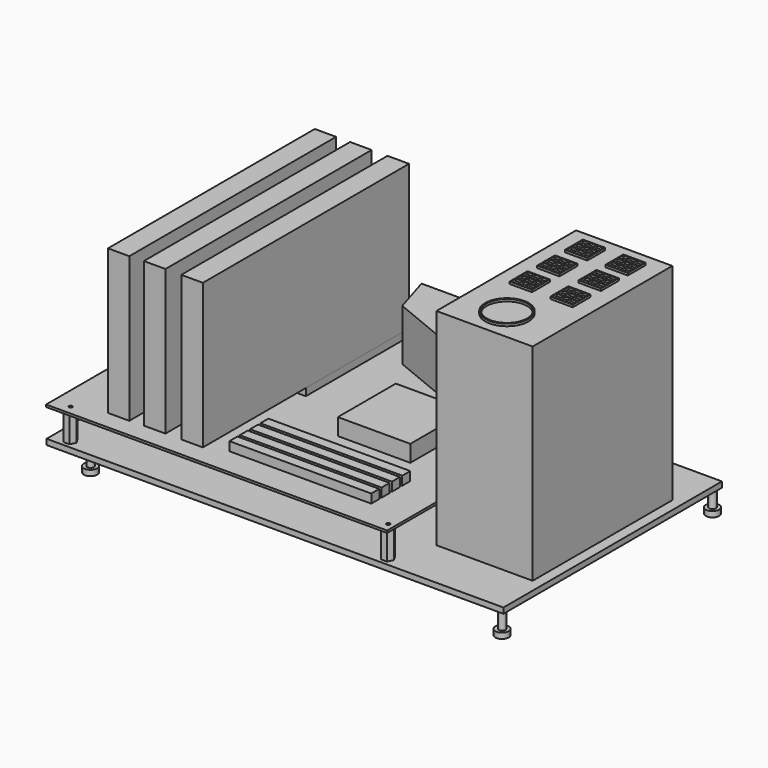
from build123d import *

# Parameters (mm, degrees)
F0_W      = 304.8
F0_H      = 245
F0_W_2    = 105
F0_W_3    = 85
F0_H_2    = 155
F1_DEPTH  = 5
F2_R      = 2
F4_DEPTH  = 25
F5_W      = 305.9651181102
F5_H      = 238.5258898139
F5_R      = 1.5110835086
F5_R_2    = 1.8546017652
F5_R_3    = 1.5453334322
F5_R_4    = 1.5864873671
F5_R_5    = 1.5329396313
F5_R_6    = 1.5189337909
F6_DEPTH  = 2
F8_DEPTH  = 46
F9_W      = 86.2980593292
F9_H      = 156.6275962591
F10_DEPTH = 185
F11_R     = 19.4404992454
F11_R_2   = 18.1570316282
F11_W     = 20
F11_H     = 20
F11_W_2   = 5.8072507381
F11_H_2   = 5.6268667936
F11_H_3   = 5.6345332414
F11_W_3   = 5.6646615267
F11_W_4   = 5.666539073
F11_W_5   = 5.6
F11_H_4   = 5.6
F11_W_6   = 5.645275116
F11_H_5   = 5.608684849
F12_DEPTH = 2
F7_W      = 10.3331357241
F7_H      = 111.6103834684
F7_W_2    = 9.9950507283
F7_H_2    = 111.5762374575
F7_H_3    = 111.7404969409
F13_DEPTH = 7
F14_W     = 19.3574428558
F14_H     = 231.2334789895
F14_W_2   = 10.3331357241
F14_H_2   = 111.6103834684
F14_W_3   = 19.1079676151
F14_H_3   = 231.8987650797
F15_DEPTH = 130
F7_W_3    = 65
F7_H_4    = 65
F16_DEPTH = 15
F7_W_4    = 127.2524446249
F7_H_5    = 8.9775174856
F17_DEPTH = 8
F18_R     = 3
F19_DEPTH = 15
F20_R     = 6
F21_DEPTH = 5


# Not quite as in the source:
# - a feature names something its author has since deleted; it is built from what else it names


with BuildPart() as f1:
    # F0 (on Top) → F1 (new body)
    with BuildSketch(Plane.XY):
        with Locations((-82.8795462154, -8.5489067304)):
            Rectangle(F0_W, F0_H)
        Polygon((-217.9899460981, -119.0375398017), (-216.8253733572, -121.0318073611), (-215.6608004927, -123.0260751322), (-216.8056005272, -125.0317585543), (-217.95040061, -127.0374420608), (-220.2597738008, -127.0488578615), (-222.5691463327, -127.060273659), (-223.7337190736, -125.0660060997), (-224.8982919382, -123.0717383286), (-223.7534917181, -121.0660545815), (-222.6086918209, -119.0603714), (-220.2993194058, -119.0489556031), align=None, mode=Mode.SUBTRACT)
        Polygon((-90.5598577739, -62.1443010035), (-89.4611932931, -64.1756228432), (-88.3625285496, -66.2069451687), (-89.5723726919, -68.1740775467), (-90.7822169912, -70.14121018), (-93.0907256892, -70.0770206068), (-95.399234657, -70.0128310261), (-96.4978992478, -67.9815089828), (-97.5965638812, -65.9501868608), (-96.386719739, -63.9830544828), (-95.1768754397, -62.0159218495), (-92.8683667417, -62.0801114227), align=None, mode=Mode.SUBTRACT)
        Polygon((68.33831607, -120.4494335332), (68.5094554206, -122.7524848222), (68.6805947525, -125.0555358592), (66.7716636058, -126.3552724604), (64.862732467, -127.6550090563), (62.7826618455, -126.6516944255), (60.7025914991, -125.6483799275), (60.5314521485, -123.3453286385), (60.3603128167, -121.0422776016), (62.2692441546, -119.7425408701), (64.1781751021, -118.4428044045), (66.2582453863, -119.4461188725), align=None, mode=Mode.SUBTRACT)
        Polygon((66.8298548613, -49.0489067304), (67.9845552805, -51.048906524), (69.1392559381, -53.0489067304), (67.9845553961, -55.0489067366), (66.8298548613, -57.0489067304), (64.5204537846, -57.0489067304), (62.2110527078, -57.0489067304), (61.0563521016, -55.0489066128), (59.9016516311, -53.0489067304), (61.056352173, -51.0489067242), (62.2110527078, -49.0489067304), (64.5204537846, -49.0489067304), align=None, mode=Mode.SUBTRACT)
        Polygon((-214.9167182465, 106.9143115381), (-213.840469393, 104.871024627), (-212.7642204714, 102.8277375865), (-213.9956343223, 100.8740354331), (-215.2270484403, 98.9203328559), (-217.5347112225, 99.0099174629), (-219.8423741843, 99.0995020768), (-220.9186230378, 101.1427889879), (-221.9948719595, 103.1860760283), (-220.7634577856, 105.1397786942), (-219.5320439906, 107.093480759), (-217.2243815961, 107.003896167), align=None, mode=Mode.SUBTRACT)
        Polygon((-90.6970964333, 107.0223465499), (-89.5289724143, 105.0301567779), (-88.3608485, 103.0379671844), (-89.5020735318, 101.0302470656), (-90.6432982822, 99.022527442), (-92.9526471492, 99.0069972534), (-95.2619959976, 98.991467065), (-96.4301198271, 100.9836565138), (-97.5982439308, 102.9758464304), (-96.4570190841, 104.9835662237), (-95.3157941487, 106.9912861729), (-93.0064452817, 107.0068163614), align=None, mode=Mode.SUBTRACT)
        Polygon((66.8699328729, 82.7181310753), (67.9002257868, 81.0905187095), (68.9305187879, 79.462906206), (68.3003771909, 77.6425906742), (67.6702358065, 75.8222757565), (65.8541689997, 75.1799921406), (64.0381027187, 74.5377087107), (62.4036458006, 75.5571097754), (60.7691898217, 76.5765102543), (60.5471225276, 78.4899656062), (60.3250552006, 80.4034212412), (61.6825983651, 81.770060566), (63.0401412837, 83.1366996433), (64.9550370207, 82.9274153656), align=None, mode=Mode.SUBTRACT)
        with Locations((122.0204537846, -8.5489067304)):
            Rectangle(F0_W_2, F0_H)
        with Locations((122.0204537846, -8.5489067304)):
            Rectangle(F0_W_3, F0_H_2, mode=Mode.SUBTRACT)
        with BuildLine():
            ThreePointArc((62.2692441546, -119.7425408701), (64.2240317575, -119.0599051032), (66.2582453863, -119.4461188725))
            Line((66.2582453863, -119.4461188725), (64.1781751021, -118.4428044045))
            Line((64.1781751021, -118.4428044045), (62.2692441546, -119.7425408701))
        make_face()
        with BuildLine():
            ThreePointArc((60.5314521485, -123.3453286385), (60.9176661018, -121.3111147656), (62.2692441546, -119.7425408701))
            Line((62.2692441546, -119.7425408701), (60.3603128167, -121.0422776016))
            Line((60.3603128167, -121.0422776016), (60.5314521485, -123.3453286385))
        make_face()
        with BuildLine():
            Line((64.862732467, -127.6550090563), (66.7716636058, -126.3552724604))
            ThreePointArc((66.7716636058, -126.3552724604), (64.8168757402, -127.0379083629), (62.7826618455, -126.6516944255))
            Line((62.7826618455, -126.6516944255), (64.862732467, -127.6550090563))
        make_face()
        with BuildLine():
            ThreePointArc((68.5094554206, -122.7524848222), (68.5177032479, -122.9005937913), (68.5204537846, -123.0489067304))
            ThreePointArc((68.5204537846, -123.0489067304), (68.0563298631, -124.9190886353), (66.7716636058, -126.3552724604))
            Line((66.7716636058, -126.3552724604), (68.6805947525, -125.0555358592))
            Line((68.6805947525, -125.0555358592), (68.5094554206, -122.7524848222))
        make_face()
        with BuildLine():
            Line((60.7025914991, -125.6483799275), (62.7826618455, -126.6516944255))
            ThreePointArc((62.7826618455, -126.6516944255), (61.2140879787, -125.3001164402), (60.5314521485, -123.3453286385))
            Line((60.5314521485, -123.3453286385), (60.7025914991, -125.6483799275))
        make_face()
        with BuildLine():
            ThreePointArc((66.2582453863, -119.4461188725), (67.8268194851, -120.7976968657), (68.5094554206, -122.7524848222))
            Line((68.5094554206, -122.7524848222), (68.33831607, -120.4494335332))
            Line((68.33831607, -120.4494335332), (66.2582453863, -119.4461188725))
        make_face()
        with BuildLine():
            ThreePointArc((-92.8683667417, -62.0801114227), (-90.8840347309, -62.6713924621), (-89.4611932931, -64.1756228432))
            Line((-89.4611932931, -64.1756228432), (-90.5598577739, -62.1443010035))
            Line((-90.5598577739, -62.1443010035), (-92.8683667417, -62.0801114227))
        make_face()
        with BuildLine():
            ThreePointArc((-96.386719739, -63.9830544828), (-94.8824892694, -62.5602130289), (-92.8683667417, -62.0801114227))
            Line((-92.8683667417, -62.0801114227), (-95.1768754397, -62.0159218495))
            Line((-95.1768754397, -62.0159218495), (-96.386719739, -63.9830544828))
        make_face()
        with BuildLine():
            ThreePointArc((-96.4978992478, -67.9815089828), (-96.9780008064, -65.9673865034), (-96.386719739, -63.9830544828))
            Line((-96.386719739, -63.9830544828), (-97.5965638812, -65.9501868608))
            Line((-97.5965638812, -65.9501868608), (-96.4978992478, -67.9815089828))
        make_face()
        with BuildLine():
            Line((-95.399234657, -70.0128310261), (-93.0907256892, -70.0770206068))
            ThreePointArc((-93.0907256892, -70.0770206068), (-95.0750577985, -69.4857395068), (-96.4978992478, -67.9815089828))
            Line((-96.4978992478, -67.9815089828), (-95.399234657, -70.0128310261))
        make_face()
        with BuildLine():
            Line((-90.7822169912, -70.14121018), (-89.5723726919, -68.1740775467))
            ThreePointArc((-89.5723726919, -68.1740775467), (-91.0766031615, -69.5969190007), (-93.0907256892, -70.0770206068))
            Line((-93.0907256892, -70.0770206068), (-90.7822169912, -70.14121018))
        make_face()
        with BuildLine():
            ThreePointArc((-89.4611932931, -64.1756228432), (-89.1018270605, -65.0970905156), (-88.9795462154, -66.0785660148))
            ThreePointArc((-88.9795462154, -66.0785660148), (-89.1306051861, -67.1674429375), (-89.5723726919, -68.1740775467))
            Line((-89.5723726919, -68.1740775467), (-88.3625285496, -66.2069451687))
            Line((-88.3625285496, -66.2069451687), (-89.4611932931, -64.1756228432))
        make_face()
        with BuildLine():
            Line((-217.95040061, -127.0374420608), (-216.8056005272, -125.0317585543))
            ThreePointArc((-216.8056005272, -125.0317585543), (-218.2624470732, -126.5030797212), (-220.2597738008, -127.0488578615))
            Line((-220.2597738008, -127.0488578615), (-217.95040061, -127.0374420608))
        make_face()
        with BuildLine():
            ThreePointArc((-216.8253733572, -121.0318073611), (-216.4184135168, -122.0040841217), (-216.2795462154, -123.0489067304))
            ThreePointArc((-216.2795462154, -123.0489067304), (-216.4132959162, -124.0746301939), (-216.8056005272, -125.0317585543))
            Line((-216.8056005272, -125.0317585543), (-215.6608004927, -123.0260751322))
            Line((-215.6608004927, -123.0260751322), (-216.8253733572, -121.0318073611))
        make_face()
        with BuildLine():
            ThreePointArc((-220.2993194058, -119.0489556031), (-218.2966945964, -119.5749609253), (-216.8253733572, -121.0318073611))
            Line((-216.8253733572, -121.0318073611), (-217.9899460981, -119.0375398017))
            Line((-217.9899460981, -119.0375398017), (-220.2993194058, -119.0489556031))
        make_face()
        with BuildLine():
            ThreePointArc((-223.7534917181, -121.0660545815), (-222.296645531, -119.5947338408), (-220.2993194058, -119.0489556031))
            Line((-220.2993194058, -119.0489556031), (-222.6086918209, -119.0603714))
            Line((-222.6086918209, -119.0603714), (-223.7534917181, -121.0660545815))
        make_face()
        with BuildLine():
            ThreePointArc((-223.7337190736, -125.0660060997), (-224.2794973455, -123.0686793729), (-223.7534917181, -121.0660545815))
            Line((-223.7534917181, -121.0660545815), (-224.8982919382, -123.0717383286))
            Line((-224.8982919382, -123.0717383286), (-223.7337190736, -125.0660060997))
        make_face()
        with BuildLine():
            Line((-222.5691463327, -127.060273659), (-220.2597738008, -127.0488578615))
            ThreePointArc((-220.2597738008, -127.0488578615), (-222.2623981713, -126.5228523432), (-223.7337190736, -125.0660060997))
            Line((-223.7337190736, -125.0660060997), (-222.5691463327, -127.060273659))
        make_face()
        with BuildLine():
            ThreePointArc((-220.7634577856, 105.1397786942), (-219.2436640245, 106.5459836353), (-217.2243815961, 107.003896167))
            Line((-217.2243815961, 107.003896167), (-219.5320439906, 107.093480759))
            Line((-219.5320439906, 107.093480759), (-220.7634577856, 105.1397786942))
        make_face()
        with BuildLine():
            Line((-215.2270484403, 98.9203328559), (-213.9956343223, 100.8740354331))
            ThreePointArc((-213.9956343223, 100.8740354331), (-215.51542831, 99.4678300303), (-217.5347112225, 99.0099174629))
            Line((-217.5347112225, 99.0099174629), (-215.2270484403, 98.9203328559))
        make_face()
        with BuildLine():
            ThreePointArc((-213.840469393, 104.871024627), (-213.4964863852, 103.9670351088), (-213.3795462154, 103.0069068074))
            ThreePointArc((-213.3795462154, 103.0069068074), (-213.5366535827, 101.8968724775), (-213.9956343223, 100.8740354331))
            Line((-213.9956343223, 100.8740354331), (-212.7642204714, 102.8277375865))
            Line((-212.7642204714, 102.8277375865), (-213.840469393, 104.871024627))
        make_face()
        with BuildLine():
            ThreePointArc((-217.2243815961, 107.003896167), (-215.2466748623, 106.3908187139), (-213.840469393, 104.871024627))
            Line((-213.840469393, 104.871024627), (-214.9167182465, 106.9143115381))
            Line((-214.9167182465, 106.9143115381), (-217.2243815961, 107.003896167))
        make_face()
        with BuildLine():
            ThreePointArc((64.5204537846, -49.0489067304), (66.5204536814, -49.5848050557), (67.9845552805, -51.048906524))
            Line((67.9845552805, -51.048906524), (66.8298548613, -49.0489067304))
            Line((66.8298548613, -49.0489067304), (64.5204537846, -49.0489067304))
        make_face()
        with BuildLine():
            ThreePointArc((67.9845552805, -51.048906524), (68.3841570589, -52.0136304349), (68.5204537846, -53.0489067304))
            ThreePointArc((68.5204537846, -53.0489067304), (68.3841570888, -54.0841829143), (67.9845553961, -55.0489067366))
            Line((67.9845553961, -55.0489067366), (69.1392559381, -53.0489067304))
            Line((69.1392559381, -53.0489067304), (67.9845552805, -51.048906524))
        make_face()
        with BuildLine():
            Line((66.8298548613, -57.0489067304), (67.9845553961, -55.0489067366))
            ThreePointArc((67.9845553961, -55.0489067366), (66.5204537815, -56.5130083473), (64.5204537846, -57.0489067304))
            Line((64.5204537846, -57.0489067304), (66.8298548613, -57.0489067304))
        make_face()
        with BuildLine():
            Line((62.2110527078, -57.0489067304), (64.5204537846, -57.0489067304))
            ThreePointArc((64.5204537846, -57.0489067304), (62.5204537258, -56.5130083116), (61.0563521016, -55.0489066128))
            Line((61.0563521016, -55.0489066128), (62.2110527078, -57.0489067304))
        make_face()
        with BuildLine():
            ThreePointArc((61.0563521016, -55.0489066128), (60.5204537846, -53.0489066589), (61.056352173, -51.0489067242))
            Line((61.056352173, -51.0489067242), (59.9016516311, -53.0489067304))
            Line((59.9016516311, -53.0489067304), (61.0563521016, -55.0489066128))
        make_face()
        with BuildLine():
            ThreePointArc((61.056352173, -51.0489067242), (62.5204537877, -49.5848051135), (64.5204537846, -49.0489067304))
            Line((64.5204537846, -49.0489067304), (62.2110527078, -49.0489067304))
            Line((62.2110527078, -49.0489067304), (61.056352173, -51.0489067242))
        make_face()
        with BuildLine():
            Line((-95.2619959976, 98.991467065), (-92.9526471492, 99.0069972534))
            ThreePointArc((-92.9526471492, 99.0069972534), (-94.9562055958, 99.5294339184), (-96.4301198271, 100.9836565138))
            Line((-96.4301198271, 100.9836565138), (-95.2619959976, 98.991467065))
        make_face()
        with BuildLine():
            Line((-90.6432982822, 99.022527442), (-89.5020735318, 101.0302470656))
            ThreePointArc((-89.5020735318, 101.0302470656), (-90.9562962825, 99.5563329843), (-92.9526471492, 99.0069972534))
            Line((-92.9526471492, 99.0069972534), (-90.6432982822, 99.022527442))
        make_face()
        with BuildLine():
            ThreePointArc((-89.5289724143, 105.0301567779), (-89.119345754, 104.0551684149), (-88.9795462154, 103.0069068074))
            ThreePointArc((-88.9795462154, 103.0069068074), (-89.1123837716, 101.984627671), (-89.5020735318, 101.0302470656))
            Line((-89.5020735318, 101.0302470656), (-88.3608485, 103.0379671844))
            Line((-88.3608485, 103.0379671844), (-89.5289724143, 105.0301567779))
        make_face()
        with BuildLine():
            ThreePointArc((-93.0064452817, 107.0068163614), (-91.0028866722, 106.4843796039), (-89.5289724143, 105.0301567779))
            Line((-89.5289724143, 105.0301567779), (-90.6970964333, 107.0223465499))
            Line((-90.6970964333, 107.0223465499), (-93.0064452817, 107.0068163614))
        make_face()
        with BuildLine():
            ThreePointArc((-96.4570190841, 104.9835662237), (-95.0027963098, 106.4574805359), (-93.0064452817, 107.0068163614))
            Line((-93.0064452817, 107.0068163614), (-95.3157941487, 106.9912861729))
            Line((-95.3157941487, 106.9912861729), (-96.4570190841, 104.9835662237))
        make_face()
        with BuildLine():
            ThreePointArc((-96.4301198271, 100.9836565138), (-96.9794557682, 102.9800075515), (-96.4570190841, 104.9835662237))
            Line((-96.4570190841, 104.9835662237), (-97.5982439308, 102.9758464304))
            Line((-97.5982439308, 102.9758464304), (-96.4301198271, 100.9836565138))
        make_face()
        with BuildLine():
            Line((-219.8423741843, 99.0995020768), (-217.5347112225, 99.0099174629))
            ThreePointArc((-217.5347112225, 99.0099174629), (-219.5124177327, 99.6229950044), (-220.9186230378, 101.1427889879))
            Line((-220.9186230378, 101.1427889879), (-219.8423741843, 99.0995020768))
        make_face()
        with BuildLine():
            ThreePointArc((-220.9186230378, 101.1427889879), (-221.376535551, 103.1620720453), (-220.7634577856, 105.1397786942))
            Line((-220.7634577856, 105.1397786942), (-221.9948719595, 103.1860760283))
            Line((-221.9948719595, 103.1860760283), (-220.9186230378, 101.1427889879))
        make_face()
        with BuildLine():
            ThreePointArc((61.6825983651, 81.770060566), (63.1867383615, 82.722194325), (64.9550370207, 82.9274153656))
            Line((64.9550370207, 82.9274153656), (63.0401412837, 83.1366996433))
            Line((63.0401412837, 83.1366996433), (61.6825983651, 81.770060566))
        make_face()
        with BuildLine():
            ThreePointArc((60.5471225276, 78.4899656062), (60.7405302771, 80.259595573), (61.6825983651, 81.770060566))
            Line((61.6825983651, 81.770060566), (60.3250552006, 80.4034212412))
            Line((60.3250552006, 80.4034212412), (60.5471225276, 78.4899656062))
        make_face()
        with BuildLine():
            Line((60.7691898217, 76.5765102543), (62.4036458006, 75.5571097754))
            ThreePointArc((62.4036458006, 75.5571097754), (61.1406816288, 76.8116680722), (60.5471225276, 78.4899656062))
            Line((60.5471225276, 78.4899656062), (60.7691898217, 76.5765102543))
        make_face()
        with BuildLine():
            Line((67.6702358065, 75.8222757565), (68.3003771909, 77.6425906742))
            ThreePointArc((68.3003771909, 77.6425906742), (67.3583091142, 76.1321258828), (65.8541689997, 75.1799921406))
            Line((65.8541689997, 75.1799921406), (67.6702358065, 75.8222757565))
        make_face()
        with BuildLine():
            ThreePointArc((67.9002257868, 81.0905187095), (68.3622689811, 80.0648508714), (68.5204537846, 78.9510932696))
            ThreePointArc((68.5204537846, 78.9510932696), (68.4650509519, 78.2876528523), (68.3003771909, 77.6425906742))
            Line((68.3003771909, 77.6425906742), (68.9305187879, 79.462906206))
            Line((68.9305187879, 79.462906206), (67.9002257868, 81.0905187095))
        make_face()
        with BuildLine():
            ThreePointArc((64.9550370207, 82.9274153656), (66.6372612398, 82.3450770936), (67.9002257868, 81.0905187095))
            Line((67.9002257868, 81.0905187095), (66.8699328729, 82.7181310753))
            Line((66.8699328729, 82.7181310753), (64.9550370207, 82.9274153656))
        make_face()
        with BuildLine():
            Line((64.0381027187, 74.5377087107), (65.8541689997, 75.1799921406))
            ThreePointArc((65.8541689997, 75.1799921406), (64.0858700772, 74.9747712252), (62.4036458006, 75.5571097754))
            Line((62.4036458006, 75.5571097754), (64.0381027187, 74.5377087107))
        make_face()
    extrude(amount=F1_DEPTH)

    # F2
    f2_edges = [f1.edges().sort_by_distance(p)[0] for p in [
        (79.520454, 68.951093, 2.5),
        (164.520454, 68.951093, 2.5),
        (164.520454, -86.048907, 2.5),
    ]]
    fillet(f2_edges, radius=F2_R)

    # F3 (on face) → F4 (join)
    with BuildSketch(Plane.XY.offset(5)):
        Polygon((-90.2990372465, -70.0709680402), (-88.2610856011, -67.0062144912), (-88.98714419, -63.3980570458), (-92.051897739, -61.3601054004), (-95.6600551844, -62.0861639894), (-97.6980068298, -65.1509175383), (-96.9719482408, -68.7590749837), (-93.9071946918, -70.7970266291), align=None)
        Polygon((67.0801376551, 74.6096194594), (69.5601223293, 78.997107622), (67.0004384588, 83.3385814322), (61.9607699141, 83.2925670798), (59.4807852398, 78.9050789172), (62.0404691103, 74.563605107), align=None)
        Polygon((-90.3999404703, 98.6316435523), (-87.9006542157, 103.0532792869), (-90.4802599609, 107.428542542), (-95.5591519606, 107.3821700625), (-98.0584382151, 102.9605343279), (-95.47883247, 98.5852710728), align=None)
        Polygon((-214.756649224, 98.3596471188), (-212.0434527714, 102.9547723892), (-214.6663497628, 107.6020320778), (-220.0024432068, 107.654166496), (-222.7156396594, 103.0590412257), (-220.0927426681, 98.4117815371), align=None)
        Polygon((-217.554516124, -127.5639243289), (-215.0069112309, -122.9464702443), (-217.7319413223, -118.4314526458), (-223.0045763069, -118.5338891319), (-225.5521812, -123.1513432164), (-222.8271511085, -127.6663608149), align=None)
        Polygon((67.2471588363, -127.5666995185), (69.796329634, -122.946407281), (67.0696245822, -118.4286144929), (61.7937487328, -118.5311139423), (59.2445779351, -123.1514061798), (61.9712829869, -127.6691989679), align=None)
        Polygon((67.1103639098, -57.4578932326), (69.633703163, -53.0104720195), (67.0437930378, -48.6014855173), (61.9305436593, -48.6399202282), (59.4072044061, -53.0873414413), (61.9971145314, -57.4963279435), align=None)
    extrude(amount=F4_DEPTH)

    # F5 (on face) → F6 (join)
    with BuildSketch(Plane.XY.offset(30)):
        with Locations((-82.6468206942, -11.9386427104)):
            Rectangle(F5_W, F5_H)
        with Locations((-220.1107740402, -122.9654997587)):
            Circle(F5_R, mode=Mode.SUBTRACT)
        with Locations((-92.8357765079, -65.9862458706)):
            Circle(F5_R_2, mode=Mode.SUBTRACT)
        with Locations((64.6875500679, -122.9429468513)):
            Circle(F5_R_3, mode=Mode.SUBTRACT)
        with Locations((64.6881014109, -52.9459677637)):
            Circle(F5_R_4, mode=Mode.SUBTRACT)
        with Locations((-217.2289043665, 103.1133905053)):
            Circle(F5_R_5, mode=Mode.SUBTRACT)
        with Locations((-92.8357765079, 103.1493768096)):
            Circle(F5_R_2, mode=Mode.SUBTRACT)
        with Locations((64.6757036448, 79.0747404099)):
            Circle(F5_R_6, mode=Mode.SUBTRACT)
    extrude(amount=F6_DEPTH)

    # F7 (on face) → F8 (join)
    with BuildSketch(Plane.XY.offset(32)):
        Polygon((70.3357383609, 94.1896761107), (70.3357383609, 107.3243021965), (-89.6642616391, 107.3243021965), (-79.1051834822, 72.5357756019), (-17.7721679211, 47.3243021965), (57.1893751621, 75.0132724643), align=None)
    extrude(amount=F8_DEPTH)

    # F9 (on face) → F10 (join)
    with BuildSketch(Plane.XY.offset(5)):
        with Locations((122.0248155296, -8.2937665284)):
            Rectangle(F9_W, F9_H)
    extrude(amount=F10_DEPTH)

    # F11 (on face) → F12 (join)
    with BuildSketch(Plane.XY.offset(190)):
        with Locations((119.7929605842, -58.7127767503)):
            Circle(F11_R)
        with Locations((119.7929605842, -58.7127767503)):
            Circle(F11_R_2, mode=Mode.SUBTRACT)
        with Locations((139.9310624599, -12.6137597056)):
            Rectangle(F11_W, F11_H)
        with Locations((133.6714923382, -19.2763534307)):
            Rectangle(F11_W_2, F11_H_2, mode=Mode.SUBTRACT)
        with Locations((133.6714923382, -12.9285277799)):
            Rectangle(F11_W_2, F11_H_3, mode=Mode.SUBTRACT)
        with Locations((140.0674507022, -19.2763534307)):
            Rectangle(F11_W_3, F11_H_2, mode=Mode.SUBTRACT)
        with Locations((140.066511929, -12.9285277799)):
            Rectangle(F11_W_4, F11_H_3, mode=Mode.SUBTRACT)
        with Locations((146.3399502516, -19.2629200339)):
            Rectangle(F11_W_5, F11_H_4, mode=Mode.SUBTRACT)
        with Locations((146.3625878096, -12.9285277799)):
            Rectangle(F11_W_6, F11_H_3, mode=Mode.SUBTRACT)
        with Locations((133.6714923382, -6.4445987809)):
            Rectangle(F11_W_2, F11_H_5, mode=Mode.SUBTRACT)
        with Locations((140.066511929, -6.4445987809)):
            Rectangle(F11_W_4, F11_H_5, mode=Mode.SUBTRACT)
        with Locations((146.3625878096, -6.4445987809)):
            Rectangle(F11_W_6, F11_H_5, mode=Mode.SUBTRACT)
        with Locations((139.9310624599, 19.0166625364)):
            Rectangle(F11_W, F11_H)
        with Locations((133.6714923382, 12.3540688112)):
            Rectangle(F11_W_2, F11_H_2, mode=Mode.SUBTRACT)
        with Locations((133.6714923382, 18.7018944621)):
            Rectangle(F11_W_2, F11_H_3, mode=Mode.SUBTRACT)
        with Locations((140.0674507022, 12.3540688112)):
            Rectangle(F11_W_3, F11_H_2, mode=Mode.SUBTRACT)
        with Locations((140.066511929, 18.7018944621)):
            Rectangle(F11_W_4, F11_H_3, mode=Mode.SUBTRACT)
        with Locations((146.3399502516, 12.367502208)):
            Rectangle(F11_W_5, F11_H_4, mode=Mode.SUBTRACT)
        with Locations((146.3625878096, 18.7018944621)):
            Rectangle(F11_W_6, F11_H_3, mode=Mode.SUBTRACT)
        with Locations((133.6714923382, 25.185823461)):
            Rectangle(F11_W_2, F11_H_5, mode=Mode.SUBTRACT)
        with Locations((140.066511929, 25.185823461)):
            Rectangle(F11_W_4, F11_H_5, mode=Mode.SUBTRACT)
        with Locations((146.3625878096, 25.185823461)):
            Rectangle(F11_W_6, F11_H_5, mode=Mode.SUBTRACT)
        with Locations((139.9310624599, 49.1166694462)):
            Rectangle(F11_W, F11_H)
        with Locations((133.6714923382, 42.454075721)):
            Rectangle(F11_W_2, F11_H_2, mode=Mode.SUBTRACT)
        with Locations((133.6714923382, 48.8019013719)):
            Rectangle(F11_W_2, F11_H_3, mode=Mode.SUBTRACT)
        with Locations((133.6714923382, 55.2858303708)):
            Rectangle(F11_W_2, F11_H_5, mode=Mode.SUBTRACT)
        with Locations((140.0674507022, 42.454075721)):
            Rectangle(F11_W_3, F11_H_2, mode=Mode.SUBTRACT)
        with Locations((140.066511929, 48.8019013719)):
            Rectangle(F11_W_4, F11_H_3, mode=Mode.SUBTRACT)
        with Locations((140.066511929, 55.2858303708)):
            Rectangle(F11_W_4, F11_H_5, mode=Mode.SUBTRACT)
        with Locations((146.3399502516, 42.4675091179)):
            Rectangle(F11_W_5, F11_H_4, mode=Mode.SUBTRACT)
        with Locations((146.3625878096, 48.8019013719)):
            Rectangle(F11_W_6, F11_H_3, mode=Mode.SUBTRACT)
        with Locations((146.3625878096, 55.2858303708)):
            Rectangle(F11_W_6, F11_H_5, mode=Mode.SUBTRACT)
        with Locations((103.3763086796, -12.6137597056)):
            Rectangle(F11_W, F11_H)
        with Locations((97.1167385578, -19.2763534307)):
            Rectangle(F11_W_2, F11_H_2, mode=Mode.SUBTRACT)
        with Locations((97.1167385578, -12.9285277799)):
            Rectangle(F11_W_2, F11_H_3, mode=Mode.SUBTRACT)
        with Locations((103.5126969218, -19.2763534307)):
            Rectangle(F11_W_3, F11_H_2, mode=Mode.SUBTRACT)
        with Locations((103.5117581487, -12.9285277799)):
            Rectangle(F11_W_4, F11_H_3, mode=Mode.SUBTRACT)
        with Locations((109.7851964712, -19.2629200339)):
            Rectangle(F11_W_5, F11_H_4, mode=Mode.SUBTRACT)
        with Locations((109.8078340292, -12.9285277799)):
            Rectangle(F11_W_6, F11_H_3, mode=Mode.SUBTRACT)
        with Locations((97.1167385578, -6.4445987809)):
            Rectangle(F11_W_2, F11_H_5, mode=Mode.SUBTRACT)
        with Locations((103.5117581487, -6.4445987809)):
            Rectangle(F11_W_4, F11_H_5, mode=Mode.SUBTRACT)
        with Locations((109.8078340292, -6.4445987809)):
            Rectangle(F11_W_6, F11_H_5, mode=Mode.SUBTRACT)
        with Locations((103.3763086796, 18.195868772)):
            Rectangle(F11_W, F11_H)
        with Locations((97.1167385578, 11.5332750468)):
            Rectangle(F11_W_2, F11_H_2, mode=Mode.SUBTRACT)
        with Locations((97.1167385578, 17.8811006976)):
            Rectangle(F11_W_2, F11_H_3, mode=Mode.SUBTRACT)
        with Locations((97.1167385578, 24.3650296966)):
            Rectangle(F11_W_2, F11_H_5, mode=Mode.SUBTRACT)
        with Locations((103.5126969218, 11.5332750468)):
            Rectangle(F11_W_3, F11_H_2, mode=Mode.SUBTRACT)
        with Locations((103.5117581487, 17.8811006976)):
            Rectangle(F11_W_4, F11_H_3, mode=Mode.SUBTRACT)
        with Locations((103.5117581487, 24.3650296966)):
            Rectangle(F11_W_4, F11_H_5, mode=Mode.SUBTRACT)
        with Locations((109.7851964712, 11.5467084436)):
            Rectangle(F11_W_5, F11_H_4, mode=Mode.SUBTRACT)
        with Locations((109.8078340292, 17.8811006976)):
            Rectangle(F11_W_6, F11_H_3, mode=Mode.SUBTRACT)
        with Locations((109.8078340292, 24.3650296966)):
            Rectangle(F11_W_6, F11_H_5, mode=Mode.SUBTRACT)
        with Locations((103.6316773295, 49.1166694462)):
            Rectangle(F11_W, F11_H)
        with Locations((97.3721072078, 42.454075721)):
            Rectangle(F11_W_2, F11_H_2, mode=Mode.SUBTRACT)
        with Locations((97.3721072078, 48.8019013719)):
            Rectangle(F11_W_2, F11_H_3, mode=Mode.SUBTRACT)
        with Locations((97.3721072078, 55.2858303708)):
            Rectangle(F11_W_2, F11_H_5, mode=Mode.SUBTRACT)
        with Locations((103.7680655718, 42.454075721)):
            Rectangle(F11_W_3, F11_H_2, mode=Mode.SUBTRACT)
        with Locations((103.7671267986, 48.8019013719)):
            Rectangle(F11_W_4, F11_H_3, mode=Mode.SUBTRACT)
        with Locations((103.7671267986, 55.2858303708)):
            Rectangle(F11_W_4, F11_H_5, mode=Mode.SUBTRACT)
        with Locations((110.0405651212, 42.4675091179)):
            Rectangle(F11_W_5, F11_H_4, mode=Mode.SUBTRACT)
        with Locations((110.0632026792, 48.8019013719)):
            Rectangle(F11_W_6, F11_H_3, mode=Mode.SUBTRACT)
        with Locations((110.0632026792, 55.2858303708)):
            Rectangle(F11_W_6, F11_H_5, mode=Mode.SUBTRACT)
    extrude(amount=F12_DEPTH)

    # F7 (on face) → F13 (join)
    with BuildSketch(Plane.XY.offset(32)):
        with Locations((-106.5507978201, 48.0596121761)):
            Rectangle(F7_W, F7_H)
        with Locations((-139.2209939659, 48.0425391706)):
            Rectangle(F7_W_2, F7_H_2)
        with Locations((-170.837175101, 47.9604094289)):
            Rectangle(F7_W_2, F7_H_3)
    extrude(amount=F13_DEPTH)

    # F14 (on face) → F15 (join)
    with BuildSketch(Plane.XY.offset(39)):
        with Locations((-110.4673743248, -8.3440102171)):
            Rectangle(F14_W, F14_H)
        with Locations((-106.5507978201, 48.0596121761)):
            Rectangle(F14_W_2, F14_H_2, mode=Mode.SUBTRACT)
        with Locations((-144.0248191357, -8.3440102171)):
            Rectangle(F14_W, F14_H)
        with Locations((-175.8084893227, -8.6766532622)):
            Rectangle(F14_W_3, F14_H_3)
        with Locations((-106.5507978201, 48.0596121761)):
            Rectangle(F14_W_2, F14_H_2)
    extrude(amount=F15_DEPTH)

    # F7 (on face) → F16 (join)
    with BuildSketch(Plane.XY.offset(32)):
        with Locations((-13.6177974939, -8.4204699099)):
            Rectangle(F7_W_3, F7_H_4)
    extrude(amount=F16_DEPTH)

    # F7 (on face) → F17 (join)
    with BuildSketch(Plane.XY.offset(32)):
        with BuildLine():
            Line((36.2135097384, -71.6332644224), (36.2135097384, -62.6557469368))
            Line((36.2135097384, -62.6557469368), (-91.0389348865, -62.6557469368))
            Line((-91.0389348865, -62.6557469368), (-91.0389348865, -65.5269987745))
            ThreePointArc((-91.0389348865, -65.5269987745), (-90.995671436, -65.7548133051), (-90.9811747426, -65.9862458706))
            ThreePointArc((-90.9811747426, -65.9862458706), (-90.995671436, -66.2176784361), (-91.0389348865, -66.4454929667))
            Line((-91.0389348865, -66.4454929667), (-91.0389348865, -71.6332644224))
            Line((-91.0389348865, -71.6332644224), (36.2135097384, -71.6332644224))
        make_face()
        with Locations((-27.412712574, -78.7220224738)):
            Rectangle(F7_W_4, F7_H_5)
        with Locations((-27.412712574, -90.299539268)):
            Rectangle(F7_W_4, F7_H_5)
        with Locations((-27.412712574, -101.8770560622)):
            Rectangle(F7_W_4, F7_H_5)
    extrude(amount=F17_DEPTH)

    # F18 (on face) → F19 (join)
    with BuildSketch(Plane(origin=(0, 0, 0), x_dir=(1, 0, 0), z_dir=(0, 0, -1))):
        with Locations((-209.4674855471, 113.9779090881)):
            Circle(F18_R)
        with Locations((169.9112206697, 126.8104016781)):
            Circle(F18_R)
        with Locations((-203.8375139236, -95.7022756338)):
            Circle(F18_R)
        with Locations((169.8072403669, -109.2654168606)):
            Circle(F18_R)
    extrude(amount=F19_DEPTH)

    # F20 (on face) → F21 (join)
    with BuildSketch(Plane(origin=(0, 0, -15), x_dir=(1, 0, 0), z_dir=(0, 0, -1))):
        with Locations((-209.4674855471, 113.9779090881)):
            Circle(F20_R)
        with Locations((-203.81757617, -95.6871807575)):
            Circle(F20_R)
        with Locations((169.8096990585, -109.2454791069)):
            Circle(F20_R)
        with Locations((169.9013113976, 126.8288940191)):
            Circle(F20_R)
    extrude(amount=F21_DEPTH)


solid = f1.part
